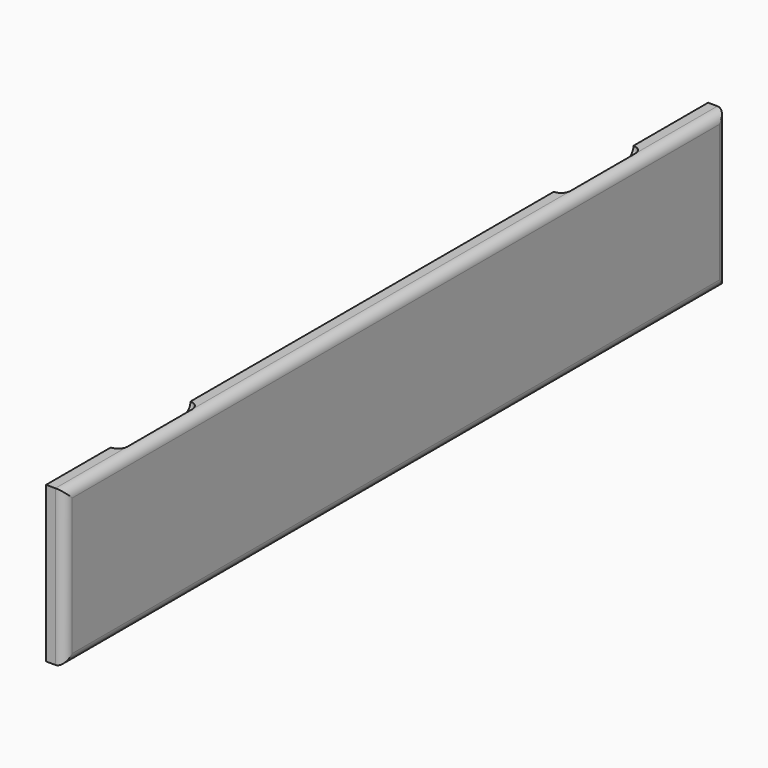
from build123d import *

# Parameters (mm, degrees)
F0_W     = 844.55
F0_H     = 158.75
F1_DEPTH = 19.05
F3_R     = 9.525
F4_DEPTH = 101.6
F5_R     = 9.52499
F7_R     = 9.525
F8_DEPTH = 101.6
F9_R     = 9.52499
F10_R    = 9.52499


# Not quite as in the source:
# - a fillet or chamfer is up to 0.001 mm smaller than in the source, because OpenCascade refuses the exact size


with BuildPart() as f1:
    # F0 (on Right) → F1 (new body)
    with BuildSketch(Plane.YZ):
        Rectangle(F0_W, F0_H)
    extrude(amount=F1_DEPTH)

    # F3 (on offset) → F4 (cut)
    with BuildSketch(Plane.XZ.offset(339.725)):
        with Locations((0, 79.375)):
            Circle(F3_R)
    extrude(amount=-F4_DEPTH, mode=Mode.SUBTRACT)

    # F5 (radius 9.525 in the source; OpenCascade refuses exactly that, so slightly less here)
    f5_edges = [f1.edges().sort_by_distance(p)[0] for p in [
        (6.735192, -339.725, 72.639808),
        (6.735192, -238.125, 72.639808),
    ]]
    fillet(f5_edges, radius=F5_R)

    # F7 (on offset) → F8 (cut)
    with BuildSketch(Plane(origin=(0, 327.025, 0), x_dir=(-1, 0, 0), z_dir=(0, 1, 0))):
        with Locations((0, 79.375)):
            Circle(F7_R)
    extrude(amount=-F8_DEPTH, mode=Mode.SUBTRACT)

    # F9 (radius 9.525 in the source; OpenCascade refuses exactly that, so slightly less here)
    f9_edges = [f1.edges().sort_by_distance(p)[0] for p in [
        (6.735192, 225.425, 72.639808),
        (6.735192, 327.025, 72.639808),
    ]]
    fillet(f9_edges, radius=F9_R)

    # F10 (radius 9.525 in the source; OpenCascade refuses exactly that, so slightly less here)
    f10_edges = [f1.edges().sort_by_distance(p)[0] for p in [
        (19.05, -422.275, 0),
        (19.05, 0, 79.375),
        (19.05, 422.275, 0),
        (19.05, 0, -79.375),
    ]]
    fillet(f10_edges, radius=F10_R)


solid = f1.part
